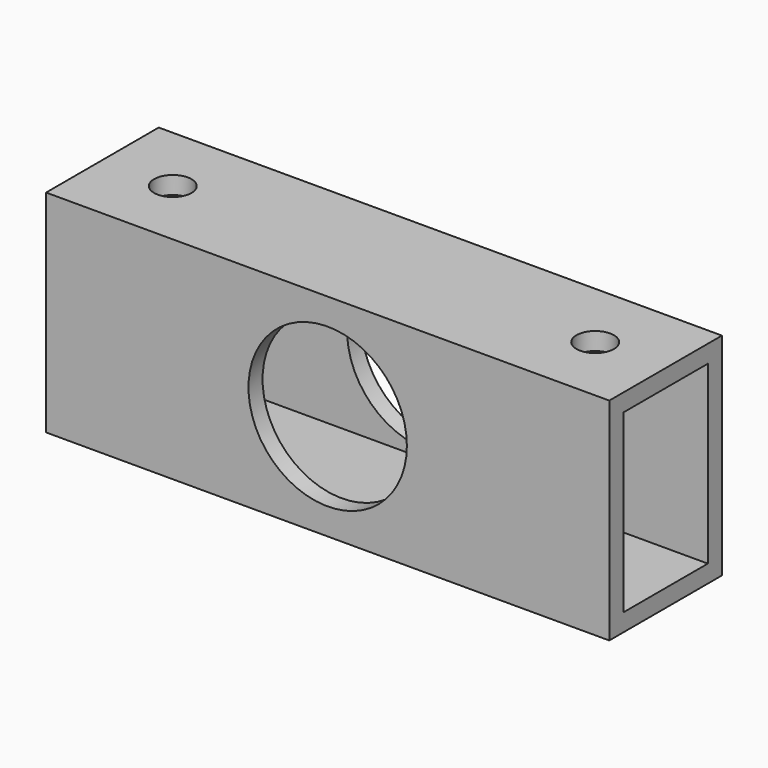
from build123d import *

# Parameters (mm, degrees)
F0_W          = 101.6
F0_H          = 25.4
F0_R          = 3.3782
F1_DEPTH      = 38.1
F2_R          = 14.2875
F3_DEPTH      = 25.4
F4_W          = 19.05
F4_H          = 31.75
F5_DEPTH      = 50.801
F5_DEPTH_BACK = 50.801


# Not quite as in the source:
# - a feature names something its author has since deleted; it is built from what else it names


with BuildPart() as f1:
    # F0 (on Top) → F1 (new body)
    with BuildSketch(Plane.XY):
        Rectangle(F0_W, F0_H)
        with Locations((-38.1, 0)):
            Circle(F0_R, mode=Mode.SUBTRACT)
        with Locations((38.1, 0)):
            Circle(F0_R, mode=Mode.SUBTRACT)
    extrude(amount=F1_DEPTH)

    # F2 (on face) → F3 (cut)
    with BuildSketch(Plane.XZ.offset(12.7)):
        with Locations((0, 19.05)):
            Circle(F2_R)
    extrude(amount=-F3_DEPTH, mode=Mode.SUBTRACT)

    # F4 (on Right) → F5 (cut, two sides)
    with BuildSketch(Plane.YZ) as f5_sk:
        with Locations((0, 19.05)):
            Rectangle(F4_W, F4_H)
    extrude(amount=-F5_DEPTH, mode=Mode.SUBTRACT)
    extrude(f5_sk.sketch, amount=F5_DEPTH_BACK, mode=Mode.SUBTRACT)


solid = f1.part
